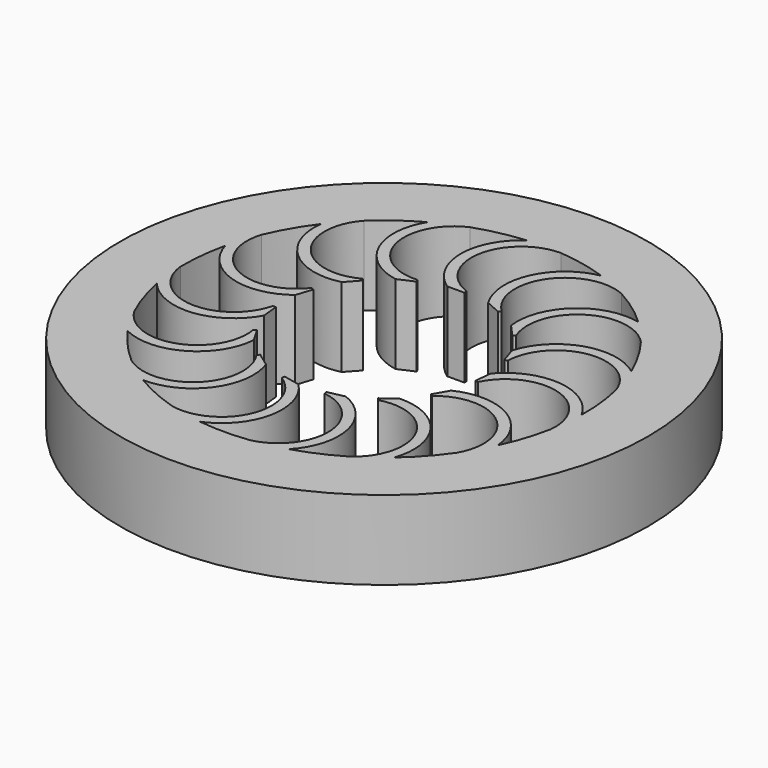
from build123d import *

# Parameters (mm, degrees)
F0_R            = 10
F0_R_2          = 7.6
F1_DEPTH        = 3
F3_DEPTH        = 3
F3_COPIES_COUNT = 15


# Not quite as in the source:
# - a pattern or mirror of a feature is missing from the dataset's text; its kind, count and spacing are read off the source's solid
# - a feature names something its author has since deleted; it is built from what else it names


with BuildPart() as f1:
    # F0 (on Top) → F1 (new body)
    with BuildSketch(Plane.XY):
        Circle(F0_R)
        Circle(F0_R_2, mode=Mode.SUBTRACT)
    extrude(amount=F1_DEPTH)

    # F2 (on Top) → F3 (join, through all)
    with BuildSketch(Plane.XY):
        with BuildLine():
            ThreePointArc((0, 3.9140510674), (-1.211569324, 6.0142199175), (0.6459488827, 7.57249959))
            ThreePointArc((0.6459488827, 7.57249959), (0, 7.6), (-0.6459488827, 7.57249959))
            ThreePointArc((-0.6459488827, 7.57249959), (-1.6403009124, 5.686249795), (-0.6459488827, 3.8))
            Line((-0.6459488827, 3.8), (0, 3.8))
            Line((0, 3.8), (0, 3.9140510674))
        make_face()
    f3 = extrude(amount=F3_DEPTH)

    # F3_copies: F3 ×15 about axis
    f3_copies_axis = Axis((0, 0, 0), (0, 0, 1))
    for i in range(1, F3_COPIES_COUNT):
        add(f3.rotate(f3_copies_axis, i * 360 / F3_COPIES_COUNT))


solid = f1.part
